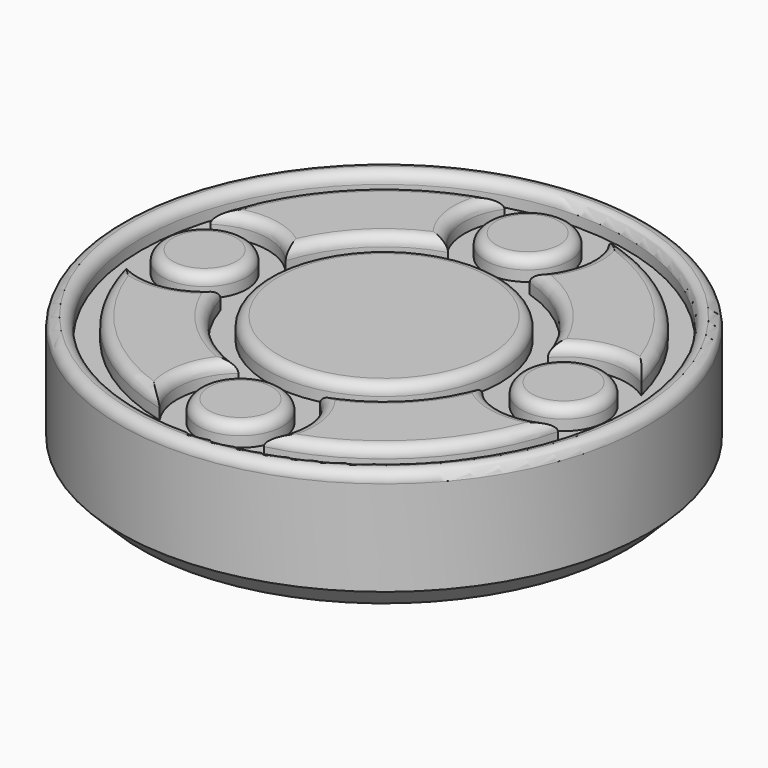
from build123d import *

# Parameters (mm, degrees)
F0_R     = 12.5
F1_DEPTH = 6
F2_R     = 11.5
F2_R_2   = 2
F2_R_3   = 5.5
F3_DEPTH = 1
F4_SIZE  = 1
F5_R     = 0.49999


# Not quite as in the source:
# - a fillet or chamfer is up to 0.001 mm smaller than in the source, because OpenCascade refuses the exact size


with BuildPart() as f1:
    # F0 (on Top) → F1 (new body)
    with BuildSketch(Plane.XY):
        Circle(F0_R)
    extrude(amount=F1_DEPTH)

    # F2 (on face) → F3 (cut)
    with BuildSketch(Plane.XY.offset(6)):
        Circle(F2_R)
        with BuildLine():
            ThreePointArc((-10.2058823529, -2.4677855251), (-8.1025492896, -2.9735556045), (-6.2058823529, -1.9331384383))
            ThreePointArc((-6.2058823529, -1.9331384383), (-4.5961940777, -4.5961940777), (-1.9331384383, -6.2058823529))
            ThreePointArc((-1.9331384383, -6.2058823529), (-2.9735556045, -8.1025492896), (-2.4677855251, -10.2058823529))
            ThreePointArc((-2.4677855251, -10.2058823529), (-7.4246212025, -7.4246212025), (-10.2058823529, -2.4677855251))
        make_face(mode=Mode.SUBTRACT)
        with Locations((0, -8.5)):
            Circle(F2_R_2, mode=Mode.SUBTRACT)
        with BuildLine():
            ThreePointArc((10.2058823529, -2.4677855251), (7.4246212025, -7.4246212025), (2.4677855251, -10.2058823529))
            ThreePointArc((2.4677855251, -10.2058823529), (2.9735556045, -8.1025492896), (1.9331384383, -6.2058823529))
            ThreePointArc((1.9331384383, -6.2058823529), (4.5961940777, -4.5961940777), (6.2058823529, -1.9331384383))
            ThreePointArc((6.2058823529, -1.9331384383), (8.1025492896, -2.9735556045), (10.2058823529, -2.4677855251))
        make_face(mode=Mode.SUBTRACT)
        with Locations((-8.5, 0)):
            Circle(F2_R_2, mode=Mode.SUBTRACT)
        with BuildLine():
            ThreePointArc((-10.2058823529, 2.4677855251), (-7.4246212025, 7.4246212025), (-2.4677855251, 10.2058823529))
            ThreePointArc((-2.4677855251, 10.2058823529), (-2.9735556045, 8.1025492896), (-1.9331384383, 6.2058823529))
            ThreePointArc((-1.9331384383, 6.2058823529), (-4.5961940777, 4.5961940777), (-6.2058823529, 1.9331384383))
            ThreePointArc((-6.2058823529, 1.9331384383), (-8.1025492896, 2.9735556045), (-10.2058823529, 2.4677855251))
        make_face(mode=Mode.SUBTRACT)
        Circle(F2_R_3, mode=Mode.SUBTRACT)
        with Locations((8.5, 0)):
            Circle(F2_R_2, mode=Mode.SUBTRACT)
        with Locations((0, 8.5)):
            Circle(F2_R_2, mode=Mode.SUBTRACT)
        with BuildLine():
            ThreePointArc((2.4677855251, 10.2058823529), (7.4246212025, 7.4246212025), (10.2058823529, 2.4677855251))
            ThreePointArc((10.2058823529, 2.4677855251), (8.1025492896, 2.9735556045), (6.2058823529, 1.9331384383))
            ThreePointArc((6.2058823529, 1.9331384383), (4.5961940777, 4.5961940777), (1.9331384383, 6.2058823529))
            ThreePointArc((1.9331384383, 6.2058823529), (2.9735556045, 8.1025492896), (2.4677855251, 10.2058823529))
        make_face(mode=Mode.SUBTRACT)
    extrude(amount=-F3_DEPTH, mode=Mode.SUBTRACT)

    # F4
    f4_edges = [f1.edges().sort_by_distance(p)[0] for p in [
        (-12.5, 0, 0),
    ]]
    chamfer(f4_edges, length=F4_SIZE)

    # F5 (radius 0.5 in the source; OpenCascade refuses exactly that, so slightly less here)
    f5_edges = [f1.edges().sort_by_distance(p)[0] for p in [
        (-12.5, 0, 6),
        (-11.5, 0, 6),
        (-2.973556, 8.102549, 6),
        (-4.596194, 4.596194, 6),
        (-8.102549, 2.973556, 6),
        (-7.424621, 7.424621, 6),
        (-10.5, 0, 6),
        (-2.973556, -8.102549, 6),
        (-7.424621, -7.424621, 6),
        (-8.102549, -2.973556, 6),
        (-4.596194, -4.596194, 6),
        (-2, -8.5, 6),
        (7.424621, -7.424621, 6),
        (2.973556, -8.102549, 6),
        (4.596194, -4.596194, 6),
        (8.102549, -2.973556, 6),
        (6.5, 0, 6),
        (2.973556, 8.102549, 6),
        (7.424621, 7.424621, 6),
        (8.102549, 2.973556, 6),
        (4.596194, 4.596194, 6),
        (-2, 8.5, 6),
        (-5.5, 0, 6),
    ]]
    fillet(f5_edges, radius=F5_R)


solid = f1.part
